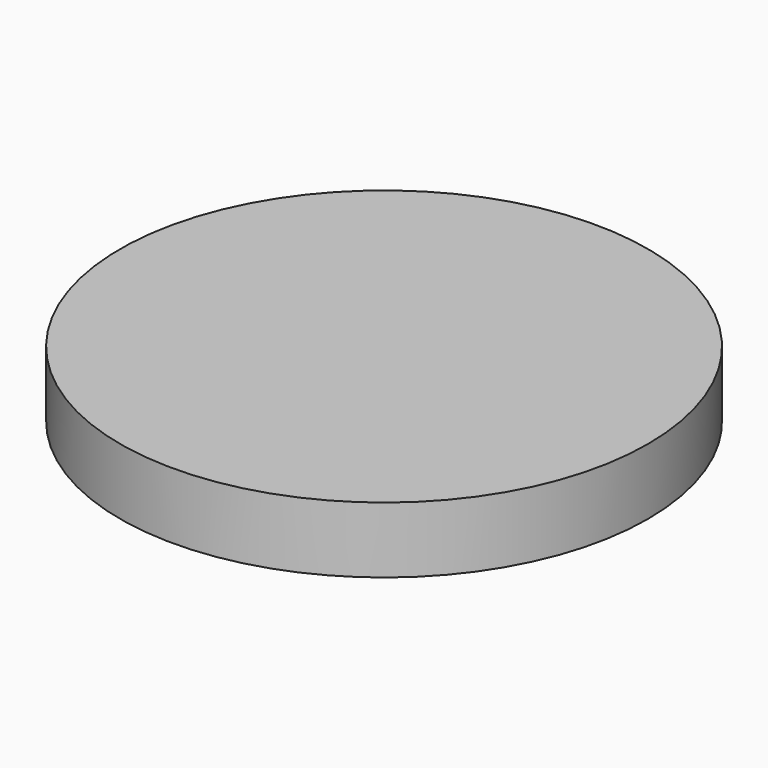
from build123d import *

# Parameters (mm, degrees)
F0_R     = 40
F1_DEPTH = 10


# Not quite as in the source:
# - the program builds the solid bodies; features that only make, move or delete a surface that nothing else refers to are left out


with BuildPart() as f1:
    # F0 (on Top) → F1 (new body)
    with BuildSketch(Plane.XY):
        Circle(F0_R)
    extrude(amount=-F1_DEPTH)


solid = f1.part
